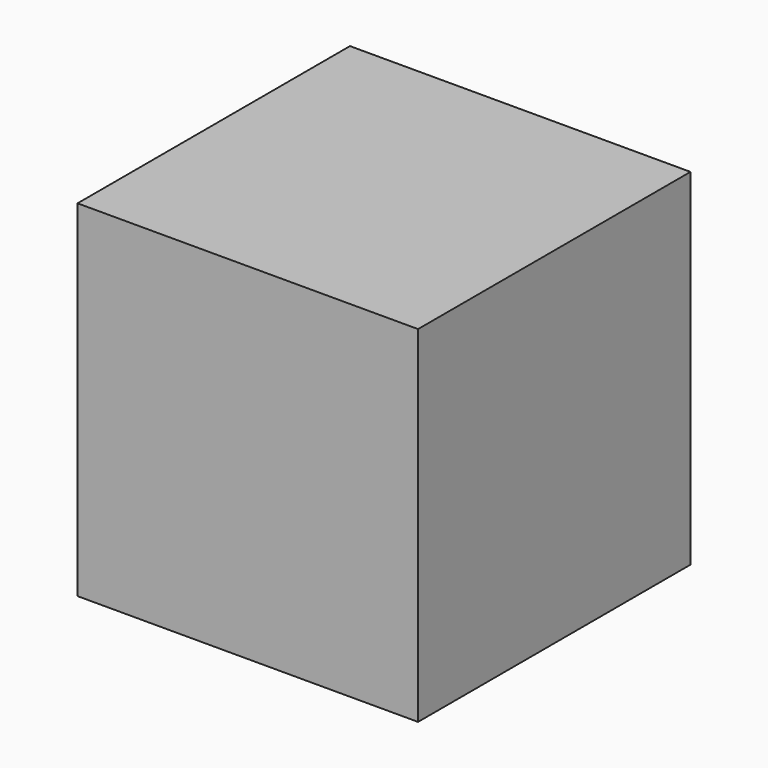
from build123d import *

# Parameters (mm, degrees)
F0_W     = 50.8
F0_H     = 50.8
F1_DEPTH = 50.8
F2_T     = -1.5875
F3_W     = 47.625
F3_H     = 0.79375
F4_DEPTH = 5.08
F7_DEPTH = 0.79375


# Not quite as in the source:
# - a length typed as a fraction of an inch, garbled in the dataset ("3 / 203.2 mm" for 3/8 in), is restored


with BuildPart() as f1:
    # F0 (on Right) → F1 (new body)
    with BuildSketch(Plane.YZ):
        with Locations((-4.0118778124, 15.742687114)):
            Rectangle(F0_W, F0_H)
    extrude(amount=F1_DEPTH)

    # F2
    f2_openings = [f1.faces().sort_by_distance(p)[0] for p in [
        (25.4, -4.011878, -9.657313),
    ]]
    offset(amount=F2_T, openings=f2_openings)

    # F3 (on face) → F4 (cut)
    with BuildSketch(Plane(origin=(0, 21.3881221876, 0), x_dir=(-1, 0, 0), z_dir=(0, 1, 0))):
        with Locations((-25.4, -9.260437886)):
            Rectangle(F3_W, F3_H)
    extrude(amount=-F4_DEPTH, mode=Mode.SUBTRACT)


with BuildPart() as f5_1:
    # F5: copy of F1
    add(f1.part)


with BuildPart() as f1_1:
    add(f1.part)

    # F7 (add): faces of the model
    f7_faces = [f1_1.faces().sort_by_distance(p)[0] for p in [
        (0.7184204897, -4.0118778124, -9.657312886),
        (25.4, 20.5943721876, -8.863562886),
    ]]
    extrude(f7_faces, amount=F7_DEPTH)


solid = f1_1.part
